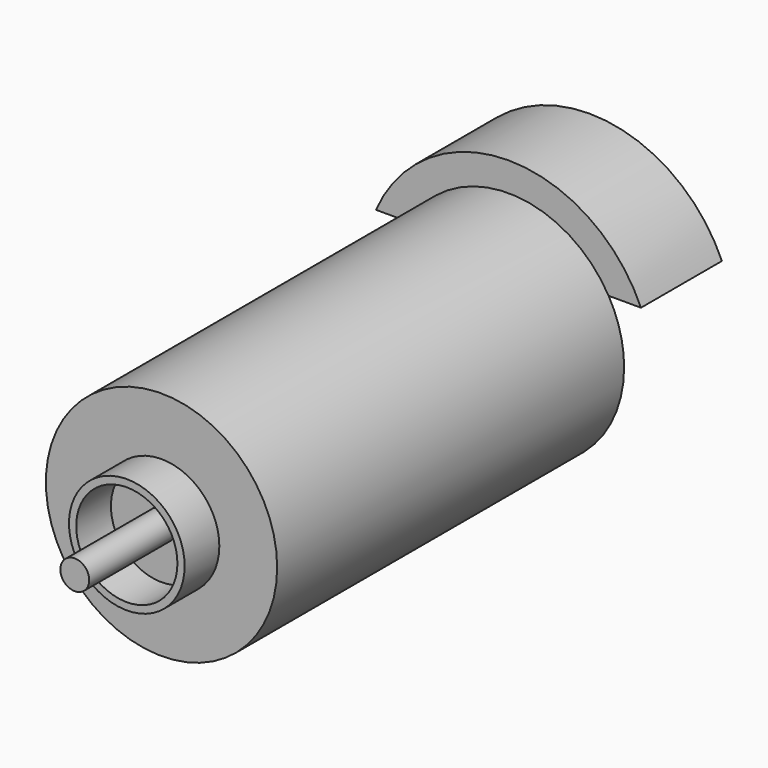
from build123d import *

# Parameters (mm, degrees)
F0_R     = 50.8
F1_DEPTH = 190.5
F2_R     = 6.35
F3_DEPTH = 47.625
F4_R     = 25.4
F4_R_2   = 22.225
F5_DEPTH = 19.05
F7_DEPTH = 44.45


# Not quite as in the source:
# - a feature names something its author has since deleted; it is built from what else it names


with BuildPart() as f1:
    # F0 (on Front) → F1 (new body)
    with BuildSketch(Plane.XZ):
        Circle(F0_R)
    extrude(amount=-F1_DEPTH)

    # F2 (on face) → F3 (join)
    with BuildSketch(Plane.XZ):
        Circle(F2_R)
    extrude(amount=F3_DEPTH)

    # F4 (on face) → F5 (join)
    with BuildSketch(Plane.XZ):
        Circle(F4_R)
        Circle(F4_R_2, mode=Mode.SUBTRACT)
    extrude(amount=F5_DEPTH)

    # F6 (on face) → F7 (join)
    with BuildSketch(Plane(origin=(0, 190.5, 0), x_dir=(-1, 0, 0), z_dir=(0, 1, 0))):
        with BuildLine():
            Line((43.9940905122, 25.4), (58.1987113259, 25.4))
            ThreePointArc((58.1987113259, 25.4), (0, 63.5), (-58.1987113259, 25.4))
            Line((-58.1987113259, 25.4), (-43.9940905122, 25.4))
            ThreePointArc((-43.9940905122, 25.4), (0, 50.8), (43.9940905122, 25.4))
        make_face()
        with BuildLine():
            Line((0, 25.4), (43.9940905122, 25.4))
            ThreePointArc((43.9940905122, 25.4), (0, 50.8), (-43.9940905122, 25.4))
            Line((-43.9940905122, 25.4), (0, 25.4))
        make_face()
    extrude(amount=F7_DEPTH)


solid = f1.part
